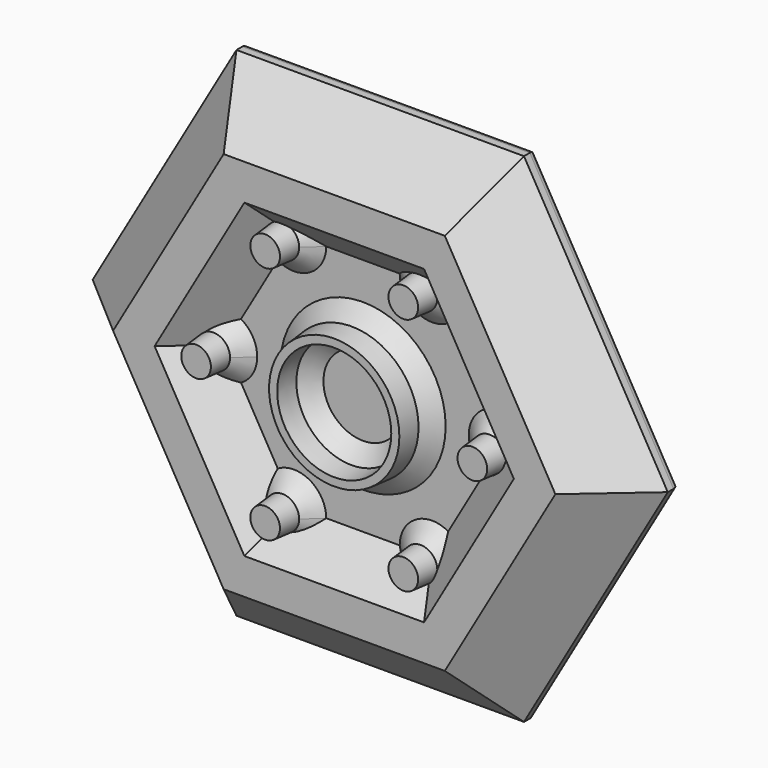
from build123d import *

# Parameters (mm, degrees)
F1_DEPTH     = 6.35
F2_SIZE      = 5.08
F4_DEPTH     = 3.175
F5_SIZE      = 3.17499
F6_R         = 0.635
F7_R         = 1.5875
F7_R_2       = 6.0325
F7_R_3       = 4.7625
F8_DEPTH     = 3.175
F8_TAPER     = 5
F9_T6_ANGLE  = 356.192567219
F9_T8_ANGLE  = 356.192567219
F9_T10_ANGLE = 238.0962831022
F9_T12_ANGLE = 118.0119864136
F9_T14_ANGLE = 178.0330528129
F9_T16_ANGLE = 178.0330528129
F9_T18_ANGLE = 118.0119864072
F9_T20_ANGLE = 238.0962831022
F9_T22_ANGLE = 356.192567219


# Not quite as in the source:
# - a fillet or chamfer that OpenCascade refuses, or shapes differently, is made with other operations: its cross-section is extruded or revolved along the edge and cut away or added
# - a fillet or chamfer is up to 0.001 mm smaller than in the source, because OpenCascade refuses the exact size


with BuildPart() as f1:
    # F0 (on Front) → F1 (new body)
    with BuildSketch(Plane.XZ):
        Polygon((-12.7, 21.9970452561), (-25.4, 0), (-12.7, -21.9970452561), (12.7, -21.9970452561), (25.4, 0), (12.7, 21.9970452561), align=None)
    extrude(amount=F1_DEPTH)

    # F2
    f2_edges = [f1.edges().sort_by_distance(p)[0] for p in [
        (0, -6.35, -21.997045),
        (19.05, -6.35, -10.998523),
        (19.05, -6.35, 10.998523),
        (0, -6.35, 21.997045),
        (-19.05, -6.35, 10.998523),
        (-19.05, -6.35, -10.998523),
    ]]
    chamfer(f2_edges, length=F2_SIZE)

    # F3 (on face) → F4 (cut)
    with BuildSketch(Plane.XZ.offset(6.35)):
        Polygon((7.9339735278, 13.7420452561), (-7.9339735278, 13.7420452561), (-15.8679470557, 0), (-7.9339735278, -13.7420452561), (7.9339735278, -13.7420452561), (15.8679470557, 0), align=None)
    extrude(amount=-F4_DEPTH, mode=Mode.SUBTRACT)

    # F5 (size 3.175 in the source; OpenCascade refuses exactly that, so slightly less here)
    f5_edges = [f1.edges().sort_by_distance(p)[0] for p in [
        (-11.90096, -3.175, 6.871023),
        (0, -3.175, 13.742045),
        (-11.90096, -3.175, -6.871023),
        (0, -3.175, -13.742045),
        (11.90096, -3.175, -6.871023),
        (11.90096, -3.175, 6.871023),
    ]]
    chamfer(f5_edges, length=F5_SIZE)

    # F6
    f6_edges = [f1.edges().sort_by_distance(p)[0] for p in [
        (19.05, 0, -10.998523),
        (19.05, 0, 10.998523),
        (0, 0, -21.997045),
        (-19.05, 0, -10.998523),
        (-19.05, 0, 10.998523),
        (0, 0, 21.997045),
    ]]
    fillet(f6_edges, radius=F6_R)

    # F7 (on face) → F8 (join)
    with BuildSketch(Plane.XZ.offset(3.175)):
        with Locations((12.2017728463, 0)):
            Circle(F7_R)
        Circle(F7_R_2)
        Circle(F7_R_3, mode=Mode.SUBTRACT)
        with Locations((6.1008864232, 10.5670452561)):
            Circle(F7_R)
        with Locations((-6.1008864232, 10.5670452561)):
            Circle(F7_R)
        with Locations((-12.2017728463, 0)):
            Circle(F7_R)
        with Locations((-6.1008864232, -10.5670452561)):
            Circle(F7_R)
        with Locations((6.1008864232, -10.5670452561)):
            Circle(F7_R)
    extrude(amount=F8_DEPTH, taper=F8_TAPER)

    # F9: chamfer of 1.27 on 11 edges, made by hand

    # F9_s1 → F9_t2 (revolve)
    with BuildSketch(Plane.XY):
        Polygon((4.8731877933, -4.4401672666), (3.4925, -3.175), (4.7625, -3.175), align=None)
    revolve(axis=Axis((0, -3.175, 0), (0, -1, 0)))

    # F9_s3 → F9_t4 (revolve)
    with BuildSketch(Plane.XY):
        Polygon((7.3025, -3.175), (5.9218122067, -4.4401672666), (6.0325, -3.175), align=None)
    revolve(axis=Axis((0, -3.175, 0), (0, -1, 0)))

    # F9_s5 → F9_t6 (revolve)
    with BuildSketch(Plane(origin=(0.0134654957, 0, -0.4051192424), x_dir=(0, 1, 0), z_dir=(0.0332200059, 0, -0.9994480633))):
        Polygon((-3.175, 15.0525382399), (-4.4401672666, 13.6718504466), (-3.175, 13.7825382399), align=None)
    revolve(axis=Axis((12.2017728463, -3.175, 0), (0, -1, 0)), revolution_arc=F9_T6_ANGLE)

    # F9_s7 → F9_t8 (revolve)
    with BuildSketch(Plane(origin=(0.3575763033, 0, -0.1908981598), x_dir=(0, 1, 0), z_dir=(0.8821574155, 0, -0.4709546626))):
        Polygon((-4.4401672666, 13.6718504466), (-3.175, 15.0525382399), (-3.175, 13.7825382399), align=None)
    revolve(axis=Axis((6.1008864232, -3.175, 10.5670452561), (0, -1, 0)), revolution_arc=F9_T8_ANGLE)

    # F9_s9 → F9_t10 (revolve)
    with BuildSketch(Plane(origin=(0.3441108974, 0, 0.2142211427), x_dir=(0, 1, 0), z_dir=(0.8489374049, 0, 0.5284934082))):
        Polygon((-3.175, 15.0525382363), (-4.4401672666, 13.671850443), (-3.175, 13.7825382363), align=None)
    revolve(axis=Axis((-6.1008864232, -3.175, 10.5670452561), (0, -1, 0)), revolution_arc=F9_T10_ANGLE)

    # F9_s11 → F9_t12 (revolve)
    with BuildSketch(Plane.XY.offset(10.5670452561)):
        Polygon((-3.2433864232, -3.175), (-4.6240742165, -4.4401672666), (-4.5133864232, -3.175), align=None)
    revolve(axis=Axis((-6.1008864232, -3.175, 10.5670452561), (0, -1, 0)), revolution_arc=F9_T12_ANGLE)

    # F9_s13 → F9_t14 (revolve)
    with BuildSketch(Plane(origin=(-0.0143744903, 0, 0.4185542247), x_dir=(0, 1, 0), z_dir=(-0.0343229619, 0, 0.9994107936))):
        Polygon((-3.175, 15.0520834832), (-4.4401672666, 13.6713956899), (-3.175, 13.7820834832), align=None)
    revolve(axis=Axis((-12.2017728463, -3.175, 0), (0, -1, 0)), revolution_arc=F9_T14_ANGLE)

    # F9_s15 → F9_t16 (revolve)
    with BuildSketch(Plane.XY):
        Polygon((-9.3442728463, -3.175), (-10.7249606396, -4.4401672666), (-10.6142728463, -3.175), align=None)
    revolve(axis=Axis((-12.2017728463, -3.175, 0), (0, -1, 0)), revolution_arc=F9_T16_ANGLE)

    # F9_s17 → F9_t18 (revolve)
    with BuildSketch(Plane(origin=(-0.3736965716, 0, 0.1987982832), x_dir=(0, 1, 0), z_dir=(-0.882849359, 0, 0.4696562672))):
        Polygon((-3.175, 15.0519286749), (-4.4401672666, 13.6712408817), (-3.175, 13.7819286749), align=None)
    revolve(axis=Axis((-6.1008864232, -3.175, -10.5670452561), (0, -1, 0)), revolution_arc=F9_T18_ANGLE)

    # F9_s19 → F9_t20 (revolve)
    with BuildSketch(Plane.XY.offset(-10.5670452561)):
        Polygon((-3.2433864232, -3.175), (-4.6240742165, -4.4401672666), (-4.5133864232, -3.175), align=None)
    revolve(axis=Axis((-6.1008864232, -3.175, -10.5670452561), (0, -1, 0)), revolution_arc=F9_T20_ANGLE)

    # F9_s21 → F9_t22 (revolve)
    with BuildSketch(Plane(origin=(-0.3441108076, 0, -0.2142210826), x_dir=(0, 1, 0), z_dir=(-0.8489374096, 0, -0.5284934007))):
        Polygon((-3.175, 15.0525382399), (-4.4401672666, 13.6718504466), (-3.175, 13.7825382399), align=None)
    revolve(axis=Axis((6.1008864232, -3.175, -10.5670452561), (0, -1, 0)), revolution_arc=F9_T22_ANGLE)


solid = f1.part
